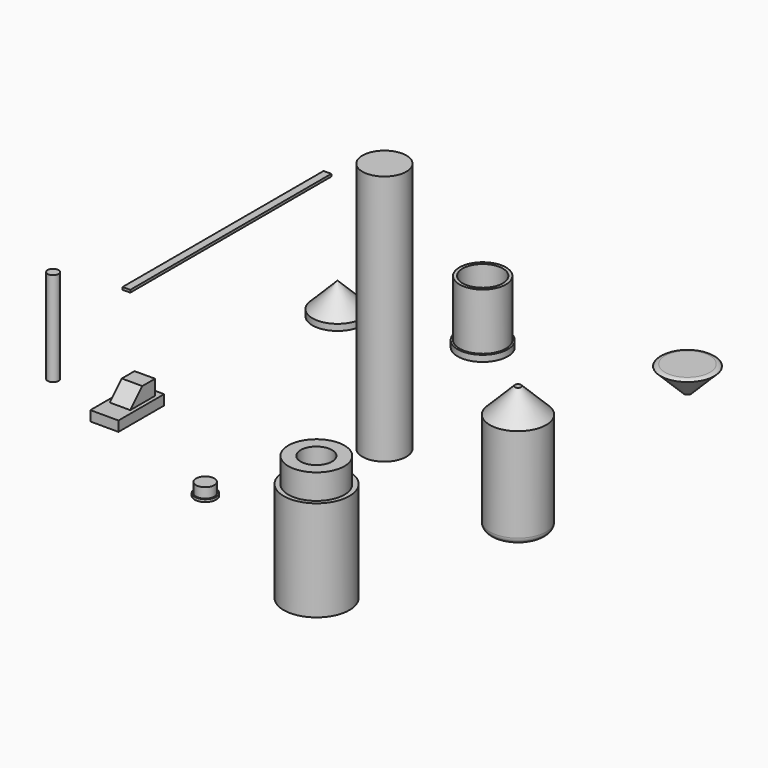
from build123d import *

# Parameters (mm, degrees)
F0_R      = 4.445
F1_DEPTH  = 50.8
F2_R      = 5.8204650715
F3_DEPTH  = 5.08
F4_R      = 1.27
F5_R      = 5.715
F6_DEPTH  = 25.4
F7_R      = 1.27
F8_SIZE   = 5.08
F10_R     = 4.6942850123
F11_DEPTH = 12.7
F12_R     = 4.064
F13_DEPTH = 6.35
F14_R     = 5.0713728951
F15_DEPTH = 1.27
F16_R     = 5.0823136585
F17_DEPTH = 6.35
F18_SIZE  = 5.08
F19_R     = 1.0996327095
F20_DEPTH = 19.05
F21_W     = 4.1527673602
F21_H     = 8.3055365831
F22_DEPTH = 5.08
F23_SIZE  = 5.07999
F24_W     = 5.6952238083
F24_H     = 11.5486495197
F25_DEPTH = 2.032
F26_W     = 1.5624314547
F26_H     = 50.8466977626
F27_DEPTH = 0.508
F28_R     = 5.6805138748
F29_DEPTH = 25.4
F31_D     = 6.35
F32_R     = 6.6491964472
F33_DEPTH = 20.32
F34_R     = 1.854860509
F35_DEPTH = 2.54
F36_R     = 2.1720678398
F37_DEPTH = 0.508
F38_R     = 1.8768217279
F39_DEPTH = 0.254


# Not quite as in the source:
# - a fillet or chamfer that OpenCascade refuses, or shapes differently, is made with other operations: its cross-section is extruded or revolved along the edge and cut away or added
# - a fillet or chamfer is up to 0.001 mm smaller than in the source, because OpenCascade refuses the exact size


with BuildPart() as f1:
    # F0 (on Top) → F1 (new body)
    with BuildSketch(Plane.XY):
        Circle(F0_R)
    extrude(amount=F1_DEPTH)


with BuildPart() as f3:
    # F2 (on Top) → F3 (new body)
    with BuildSketch(Plane.XY):
        with Locations((25.401096791, 44.9191108346)):
            Circle(F2_R)
    extrude(amount=F3_DEPTH)

    # F4
    f4_edges = [f3.edges().sort_by_distance(p)[0] for p in [
        (19.580632, 44.919111, 5.08),
    ]]
    fillet(f4_edges, radius=F4_R)

    # F9: chamfer of 5.08 on 3 edges, made by hand

    # F9_s1 → F9_t2 (revolve, cut)
    with BuildSketch(Plane.XZ.offset(-44.9191108346)):
        Polygon((31.2215618626, 5.08), (26.1415618626, 0), (31.2215618626, 0), align=None)
    revolve(axis=Axis((25.401096791, 44.9191108346, 0), (0, 0, 1)), mode=Mode.SUBTRACT)


with BuildPart() as f6:
    # F5 (on Top) → F6 (new body)
    with BuildSketch(Plane.XY):
        with Locations((33.5599295795, -8.1593608484)):
            Circle(F5_R)
    extrude(amount=F6_DEPTH)

    # F7
    f7_edges = [f6.edges().sort_by_distance(p)[0] for p in [
        (27.84493, -8.159361, 0),
    ]]
    fillet(f7_edges, radius=F7_R)

    # F8
    f8_edges = [f6.edges().sort_by_distance(p)[0] for p in [
        (29.11493, -8.159361, 0),
        (39.27493, -8.159361, 13.335),
        (27.84493, -8.159361, 1.27),
        (27.84493, -8.159361, 25.4),
    ]]
    chamfer(f8_edges, length=F8_SIZE)


with BuildPart() as f11:
    # F10 (on Top) → F11 (new body)
    with BuildSketch(Plane.XY):
        with Locations((-9.5724938437, 36.8314981461)):
            Circle(F10_R)
    extrude(amount=F11_DEPTH)

    # F12 (on face) → F13 (cut)
    with BuildSketch(Plane.XY.offset(12.7)):
        with Locations((-9.5724938437, 36.8314981461)):
            Circle(F12_R)
    extrude(amount=-F13_DEPTH, mode=Mode.SUBTRACT)

    # F14 (on face) → F15 (join)
    with BuildSketch(Plane(origin=(0, 0, 0), x_dir=(1, 0, 0), z_dir=(0, 0, -1))):
        with Locations((-9.5724938437, -36.8314981461)):
            Circle(F14_R)
    extrude(amount=-F15_DEPTH)


with BuildPart() as f17:
    # F16 (on Top) → F17 (new body)
    with BuildSketch(Plane.XY):
        with Locations((-34.1219119728, 30.7996980846)):
            Circle(F16_R)
    extrude(amount=F17_DEPTH)

    # F18
    f18_edges = [f17.edges().sort_by_distance(p)[0] for p in [
        (-39.204226, 30.799698, 6.35),
    ]]
    chamfer(f18_edges, length=F18_SIZE)


with BuildPart() as f20:
    # F19 (on Top) → F20 (new body)
    with BuildSketch(Plane.XY):
        with Locations((-55.8069758117, -14.0684247017)):
            Circle(F19_R)
    extrude(amount=F20_DEPTH)


with BuildPart() as f22:
    # F21 (on Top) → F22 (new body)
    with BuildSketch(Plane.XY):
        with Locations((-39.2436608672, -15.7113065943)):
            Rectangle(F21_W, F21_H)
    extrude(amount=F22_DEPTH)

    # F23 (size 5.08 in the source; OpenCascade refuses exactly that, so slightly less here)
    f23_edges = [f22.edges().sort_by_distance(p)[0] for p in [
        (-39.243661, -19.864075, 5.08),
    ]]
    chamfer(f23_edges, length=F23_SIZE)

    # F24 (on Top) → F25 (join)
    with BuildSketch(Plane.XY):
        with Locations((-39.2524786294, -15.9913040698)):
            Rectangle(F24_W, F24_H)
    extrude(amount=F25_DEPTH)


with BuildPart() as f27:
    # F26 (on Top) → F27 (new body)
    with BuildSketch(Plane.XY):
        with Locations((-65.4950290918, 42.0305496082)):
            Rectangle(F26_W, F26_H)
    extrude(amount=F27_DEPTH)


with BuildPart() as f29:
    # F28 (on Top) → F29 (new body)
    with BuildSketch(Plane.XY):
        with Locations((23.60156551, -46.7186421156)):
            Circle(F28_R)
    extrude(amount=F29_DEPTH)

    # F31 (through all)
    with Locations(Plane.XY.offset(25.4)):
        with Locations((23.60156551, -46.7186421156)):
            Hole(F31_D / 2)

    # F32 (on Top) → F33 (join)
    with BuildSketch(Plane.XY):
        with Locations((23.5493015498, -46.6014072299)):
            Circle(F32_R)
    extrude(amount=F33_DEPTH)


with BuildPart() as f35:
    # F34 (on Top) → F35 (new body)
    with BuildSketch(Plane.XY):
        with Locations((-11.9893560186, -30.3519330919)):
            Circle(F34_R)
    extrude(amount=F35_DEPTH)

    # F36 (on Top) → F37 (join)
    with BuildSketch(Plane.XY):
        with Locations((-12.018638663, -30.2576180547)):
            Circle(F36_R)
    extrude(amount=F37_DEPTH)

    # F38 (on face) → F39 (cut)
    with BuildSketch(Plane(origin=(0, 0, 0), x_dir=(1, 0, 0), z_dir=(0, 0, -1))):
        with Locations((-12.018638663, 30.2576180547)):
            Circle(F38_R)
    extrude(amount=-F39_DEPTH, mode=Mode.SUBTRACT)


solid = Compound([f1.part, f3.part, f6.part, f11.part, f17.part, f20.part, f22.part, f27.part, f29.part, f35.part])
